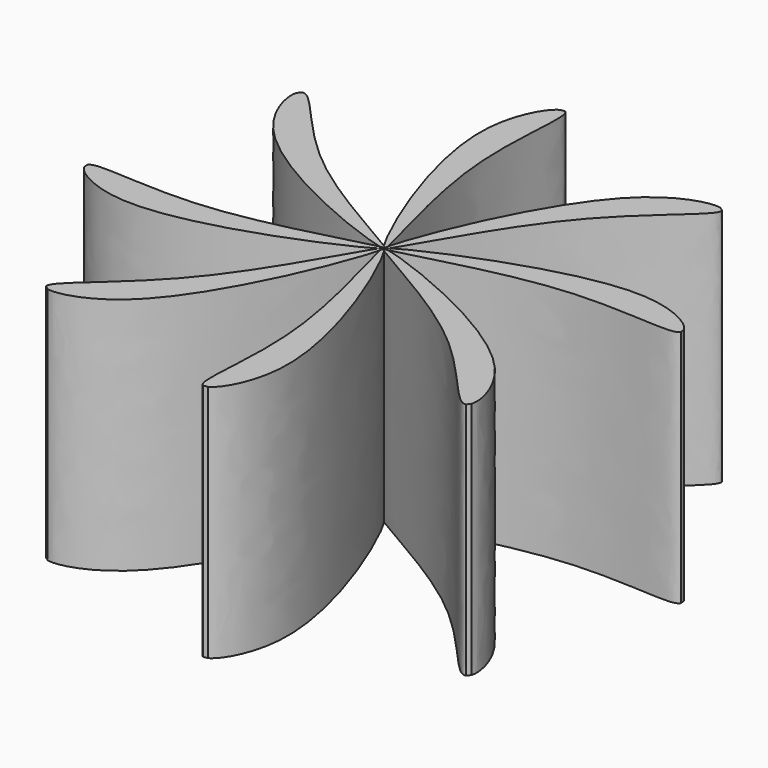
from build123d import *

# Parameters (mm, degrees)
F1_DEPTH = 12.7


with BuildPart() as f1:
    # F0 (on Top) → F1 (new body)
    with BuildSketch(Plane.XY):
        with BuildLine():
            add(Edge.make_bspline(
                [(14.3220441214, 1.8411312267), (14.1090744497, 1.3343197104), (8.7025037056, 2.6296370998), (1.1996267139, 0.1518138278), (0.2347746578, -0.0225932885)],
                knots=[0.4981451518, 0.4981451518, 0.4981451518, 0.4981451518, 0.7315463646, 0.9581958063, 0.9581958063, 0.9581958063, 0.9581958063], degree=3))
            ThreePointArc((14.3220441214, 1.8411312267), (14.3069129075, 1.9552378542), (14.2908725977, 2.0692202411))
            add(Edge.make_bspline(
                [(0.1819866201, 0.1500348851), (1.2973737053, 0.8798693546), (10.3104492256, 4.8699327901), (14.037847331, 2.5601286844), (14.2908725977, 2.0692202411)],
                knots=[0.0262614039, 0.0262614039, 0.0262614039, 0.0262614039, 0.313907198, 0.4699548858, 0.4699548858, 0.4699548858, 0.4699548858], degree=3))
            add(Edge.make_bspline(
                [(0.1819866201, 0.1500348851), (0.1337933952, 0.0805745461), (0.0944594245, 0.0309746372), (0.0645641054, 0.0035933646)],
                knots=[0.9581958063, 0.9581958063, 0.9581958063, 0.9581958063, 0.9777384816, 0.9777384816, 0.9777384816, 0.9777384816], degree=3))
            add(Edge.make_bspline(
                [(0.0645641054, 0.0035933646), (0.1066733788, 0.0010488883), (0.1638439629, -0.0077725669), (0.2347746578, -0.0225932885)],
                knots=[0.0106242136, 0.0106242136, 0.0106242136, 0.0106242136, 0.0262614039, 0.0262614039, 0.0262614039, 0.0262614039], degree=3))
        make_face()
    extrude(amount=F1_DEPTH)


with BuildPart() as f1b:
    # F0 (on Top) → F1, piece 2 (new body)
    with BuildSketch(Plane.XY):
        with BuildLine():
            ThreePointArc((11.4290908942, -8.8253381433), (11.4990770803, -8.7339531892), (11.5683325871, -8.6420132587))
            add(Edge.make_bspline(
                [(0.2347746578, -0.0225932885), (1.539543332, -0.2952201575), (10.7341510643, -3.8470260647), (11.7365413944, -8.1159726876), (11.5683325871, -8.6420132587)],
                knots=[0.0262614039, 0.0262614039, 0.0262614039, 0.0262614039, 0.313907198, 0.4699548858, 0.4699548858, 0.4699548858, 0.4699548858], degree=3))
            add(Edge.make_bspline(
                [(0.2347746578, -0.0225932885), (0.1515810249, -0.0376314091), (0.0886952756, -0.0448905236), (0.0481946092, -0.0431128243)],
                knots=[0.9581958063, 0.9581958063, 0.9581958063, 0.9581958063, 0.9777384816, 0.9777384816, 0.9777384816, 0.9777384816], degree=3))
            add(Edge.make_bspline(
                [(0.0481946092, -0.0431128243), (0.0761711456, -0.0746877935), (0.1103591424, -0.121351212), (0.1500348851, -0.1819866201)],
                knots=[0.0106242136, 0.0106242136, 0.0106242136, 0.0106242136, 0.0262614039, 0.0262614039, 0.0262614039, 0.0262614039], degree=3))
            add(Edge.make_bspline(
                [(11.4290908942, -8.8253381433), (10.9201287351, -9.0331157042), (8.0130336089, -4.2941651582), (0.9556127714, -0.7409155972), (0.1500348851, -0.1819866201)],
                knots=[0.4981451518, 0.4981451518, 0.4981451518, 0.4981451518, 0.7315463646, 0.9581958063, 0.9581958063, 0.9581958063, 0.9581958063], degree=3))
        make_face()
    extrude(amount=F1_DEPTH)


with BuildPart() as f1c:
    # F0 (on Top) → F1, piece 3 (new body)
    with BuildSketch(Plane.XY):
        with BuildLine():
            add(Edge.make_bspline(
                [(8.8253381433, 11.4290908942), (9.0331157042, 10.9201287351), (4.2941651582, 8.0130336089), (0.7409155972, 0.9556127714), (0.1819866201, 0.1500348851)],
                knots=[0.4981451518, 0.4981451518, 0.4981451518, 0.4981451518, 0.7315463646, 0.9581958063, 0.9581958063, 0.9581958063, 0.9581958063], degree=3))
            ThreePointArc((8.8253381433, 11.4290908942), (8.7339531892, 11.4990770803), (8.6420132587, 11.5683325871))
            add(Edge.make_bspline(
                [(0.0225932885, 0.2347746578), (0.2952201575, 1.539543332), (3.8470260647, 10.7341510643), (8.1159726876, 11.7365413944), (8.6420132587, 11.5683325871)],
                knots=[0.0262614039, 0.0262614039, 0.0262614039, 0.0262614039, 0.313907198, 0.4699548858, 0.4699548858, 0.4699548858, 0.4699548858], degree=3))
            add(Edge.make_bspline(
                [(0.0225932885, 0.2347746578), (0.0376314091, 0.1515810249), (0.0448905236, 0.0886952756), (0.0431128243, 0.0481946092)],
                knots=[0.9581958063, 0.9581958063, 0.9581958063, 0.9581958063, 0.9777384816, 0.9777384816, 0.9777384816, 0.9777384816], degree=3))
            add(Edge.make_bspline(
                [(0.0431128243, 0.0481946092), (0.0746877935, 0.0761711456), (0.121351212, 0.1103591424), (0.1819866201, 0.1500348851)],
                knots=[0.0106242136, 0.0106242136, 0.0106242136, 0.0106242136, 0.0262614039, 0.0262614039, 0.0262614039, 0.0262614039], degree=3))
        make_face()
    extrude(amount=F1_DEPTH)


with BuildPart() as f1d:
    # F0 (on Top) → F1, piece 4 (new body)
    with BuildSketch(Plane.XY):
        with BuildLine():
            ThreePointArc((1.8411312267, -14.3220441214), (1.9552378542, -14.3069129075), (2.0692202411, -14.2908725977))
            add(Edge.make_bspline(
                [(0.1500348851, -0.1819866201), (0.8798693546, -1.2973737053), (4.8699327901, -10.3104492256), (2.5601286844, -14.037847331), (2.0692202411, -14.2908725977)],
                knots=[0.0262614039, 0.0262614039, 0.0262614039, 0.0262614039, 0.313907198, 0.4699548858, 0.4699548858, 0.4699548858, 0.4699548858], degree=3))
            add(Edge.make_bspline(
                [(0.1500348851, -0.1819866201), (0.0805745461, -0.1337933952), (0.0309746372, -0.0944594245), (0.0035933646, -0.0645641054)],
                knots=[0.9581958063, 0.9581958063, 0.9581958063, 0.9581958063, 0.9777384816, 0.9777384816, 0.9777384816, 0.9777384816], degree=3))
            add(Edge.make_bspline(
                [(0.0035933646, -0.0645641054), (0.0010488883, -0.1066733788), (-0.0077725669, -0.1638439629), (-0.0225932885, -0.2347746578)],
                knots=[0.0106242136, 0.0106242136, 0.0106242136, 0.0106242136, 0.0262614039, 0.0262614039, 0.0262614039, 0.0262614039], degree=3))
            add(Edge.make_bspline(
                [(1.8411312267, -14.3220441214), (1.3343197104, -14.1090744497), (2.6296370998, -8.7025037056), (0.1518138278, -1.1996267139), (-0.0225932885, -0.2347746578)],
                knots=[0.4981451518, 0.4981451518, 0.4981451518, 0.4981451518, 0.7315463646, 0.9581958063, 0.9581958063, 0.9581958063, 0.9581958063], degree=3))
        make_face()
    extrude(amount=F1_DEPTH)


with BuildPart() as f1e:
    # F0 (on Top) → F1, piece 5 (new body)
    with BuildSketch(Plane.XY):
        with BuildLine():
            add(Edge.make_bspline(
                [(-1.8411312267, 14.3220441214), (-1.3343197104, 14.1090744497), (-2.6296370998, 8.7025037056), (-0.1518138278, 1.1996267139), (0.0225932885, 0.2347746578)],
                knots=[0.4981451518, 0.4981451518, 0.4981451518, 0.4981451518, 0.7315463646, 0.9581958063, 0.9581958063, 0.9581958063, 0.9581958063], degree=3))
            ThreePointArc((-1.8411312267, 14.3220441214), (-1.9552378542, 14.3069129075), (-2.0692202411, 14.2908725977))
            add(Edge.make_bspline(
                [(-0.1500348851, 0.1819866201), (-0.8798693546, 1.2973737053), (-4.8699327901, 10.3104492256), (-2.5601286844, 14.037847331), (-2.0692202411, 14.2908725977)],
                knots=[0.0262614039, 0.0262614039, 0.0262614039, 0.0262614039, 0.313907198, 0.4699548858, 0.4699548858, 0.4699548858, 0.4699548858], degree=3))
            add(Edge.make_bspline(
                [(-0.1500348851, 0.1819866201), (-0.0805745461, 0.1337933952), (-0.0309746372, 0.0944594245), (-0.0035933646, 0.0645641054)],
                knots=[0.9581958063, 0.9581958063, 0.9581958063, 0.9581958063, 0.9777384816, 0.9777384816, 0.9777384816, 0.9777384816], degree=3))
            add(Edge.make_bspline(
                [(-0.0035933646, 0.0645641054), (-0.0010488883, 0.1066733788), (0.0077725669, 0.1638439629), (0.0225932885, 0.2347746578)],
                knots=[0.0106242136, 0.0106242136, 0.0106242136, 0.0106242136, 0.0262614039, 0.0262614039, 0.0262614039, 0.0262614039], degree=3))
        make_face()
    extrude(amount=F1_DEPTH)


with BuildPart() as f1f:
    # F0 (on Top) → F1, piece 6 (new body)
    with BuildSketch(Plane.XY):
        with BuildLine():
            ThreePointArc((-8.8253381433, -11.4290908942), (-8.7339531892, -11.4990770803), (-8.6420132587, -11.5683325871))
            add(Edge.make_bspline(
                [(-0.0225932885, -0.2347746578), (-0.2952201575, -1.539543332), (-3.8470260647, -10.7341510643), (-8.1159726876, -11.7365413944), (-8.6420132587, -11.5683325871)],
                knots=[0.0262614039, 0.0262614039, 0.0262614039, 0.0262614039, 0.313907198, 0.4699548858, 0.4699548858, 0.4699548858, 0.4699548858], degree=3))
            add(Edge.make_bspline(
                [(-0.0225932885, -0.2347746578), (-0.0376314091, -0.1515810249), (-0.0448905236, -0.0886952756), (-0.0431128243, -0.0481946092)],
                knots=[0.9581958063, 0.9581958063, 0.9581958063, 0.9581958063, 0.9777384816, 0.9777384816, 0.9777384816, 0.9777384816], degree=3))
            add(Edge.make_bspline(
                [(-0.0431128243, -0.0481946092), (-0.0746877935, -0.0761711456), (-0.121351212, -0.1103591424), (-0.1819866201, -0.1500348851)],
                knots=[0.0106242136, 0.0106242136, 0.0106242136, 0.0106242136, 0.0262614039, 0.0262614039, 0.0262614039, 0.0262614039], degree=3))
            add(Edge.make_bspline(
                [(-8.8253381433, -11.4290908942), (-9.0331157042, -10.9201287351), (-4.2941651582, -8.0130336089), (-0.7409155972, -0.9556127714), (-0.1819866201, -0.1500348851)],
                knots=[0.4981451518, 0.4981451518, 0.4981451518, 0.4981451518, 0.7315463646, 0.9581958063, 0.9581958063, 0.9581958063, 0.9581958063], degree=3))
        make_face()
    extrude(amount=F1_DEPTH)


with BuildPart() as f1g:
    # F0 (on Top) → F1, piece 7 (new body)
    with BuildSketch(Plane.XY):
        with BuildLine():
            add(Edge.make_bspline(
                [(-11.4290908942, 8.8253381433), (-10.9201287351, 9.0331157042), (-8.0130336089, 4.2941651582), (-0.9556127714, 0.7409155972), (-0.1500348851, 0.1819866201)],
                knots=[0.4981451518, 0.4981451518, 0.4981451518, 0.4981451518, 0.7315463646, 0.9581958063, 0.9581958063, 0.9581958063, 0.9581958063], degree=3))
            ThreePointArc((-11.4290908942, 8.8253381433), (-11.4990770803, 8.7339531892), (-11.5683325871, 8.6420132587))
            add(Edge.make_bspline(
                [(-0.2347746578, 0.0225932885), (-1.539543332, 0.2952201575), (-10.7341510643, 3.8470260647), (-11.7365413944, 8.1159726876), (-11.5683325871, 8.6420132587)],
                knots=[0.0262614039, 0.0262614039, 0.0262614039, 0.0262614039, 0.313907198, 0.4699548858, 0.4699548858, 0.4699548858, 0.4699548858], degree=3))
            add(Edge.make_bspline(
                [(-0.2347746578, 0.0225932885), (-0.1515810249, 0.0376314091), (-0.0886952756, 0.0448905236), (-0.0481946092, 0.0431128243)],
                knots=[0.9581958063, 0.9581958063, 0.9581958063, 0.9581958063, 0.9777384816, 0.9777384816, 0.9777384816, 0.9777384816], degree=3))
            add(Edge.make_bspline(
                [(-0.0481946092, 0.0431128243), (-0.0761711456, 0.0746877935), (-0.1103591424, 0.121351212), (-0.1500348851, 0.1819866201)],
                knots=[0.0106242136, 0.0106242136, 0.0106242136, 0.0106242136, 0.0262614039, 0.0262614039, 0.0262614039, 0.0262614039], degree=3))
        make_face()
    extrude(amount=F1_DEPTH)


with BuildPart() as f1h:
    # F0 (on Top) → F1, piece 8 (new body)
    with BuildSketch(Plane.XY):
        with BuildLine():
            add(Edge.make_bspline(
                [(-0.1819866201, -0.1500348851), (-0.1337933952, -0.0805745461), (-0.0944594245, -0.0309746372), (-0.0645641054, -0.0035933646)],
                knots=[0.9581958063, 0.9581958063, 0.9581958063, 0.9581958063, 0.9777384816, 0.9777384816, 0.9777384816, 0.9777384816], degree=3))
            add(Edge.make_bspline(
                [(-0.0645641054, -0.0035933646), (-0.1066733788, -0.0010488883), (-0.1638439629, 0.0077725669), (-0.2347746578, 0.0225932885)],
                knots=[0.0106242136, 0.0106242136, 0.0106242136, 0.0106242136, 0.0262614039, 0.0262614039, 0.0262614039, 0.0262614039], degree=3))
            add(Edge.make_bspline(
                [(-14.3220441214, -1.8411312267), (-14.1090744497, -1.3343197104), (-8.7025037056, -2.6296370998), (-1.1996267139, -0.1518138278), (-0.2347746578, 0.0225932885)],
                knots=[0.4981451518, 0.4981451518, 0.4981451518, 0.4981451518, 0.7315463646, 0.9581958063, 0.9581958063, 0.9581958063, 0.9581958063], degree=3))
            ThreePointArc((-14.3220441214, -1.8411312267), (-14.3069129075, -1.9552378542), (-14.2908725977, -2.0692202411))
            add(Edge.make_bspline(
                [(-0.1819866201, -0.1500348851), (-1.2973737053, -0.8798693546), (-10.3104492256, -4.8699327901), (-14.037847331, -2.5601286844), (-14.2908725977, -2.0692202411)],
                knots=[0.0262614039, 0.0262614039, 0.0262614039, 0.0262614039, 0.313907198, 0.4699548858, 0.4699548858, 0.4699548858, 0.4699548858], degree=3))
        make_face()
    extrude(amount=F1_DEPTH)


solid = Compound([f1.part, f1b.part, f1c.part, f1d.part, f1e.part, f1f.part, f1g.part, f1h.part])
